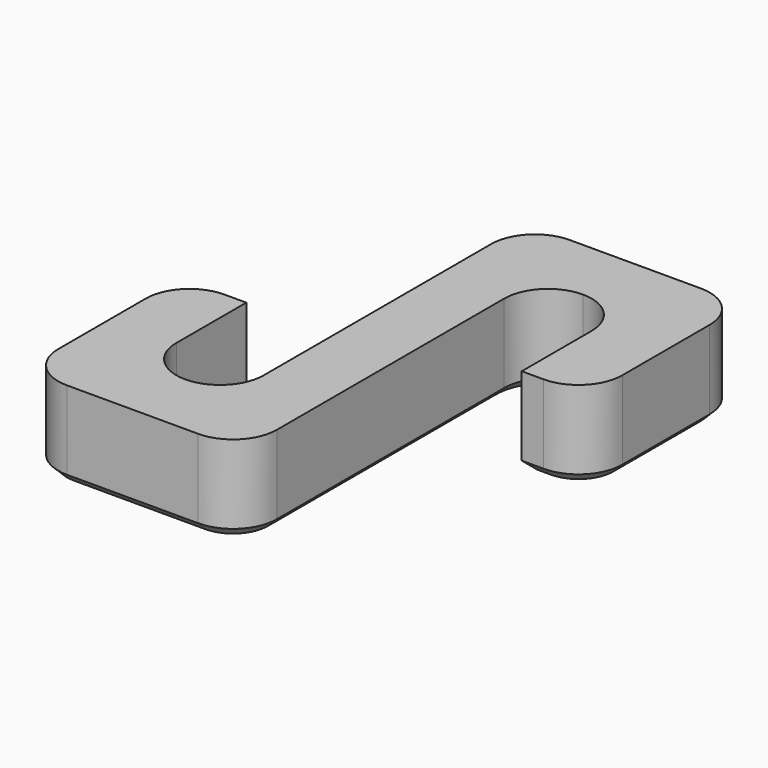
from build123d import *

# Parameters (mm, degrees)
F1_DEPTH = 2
F2_R     = 0.99999
F3_SIZE  = 0.2


# Not quite as in the source:
# - a fillet or chamfer is up to 0.001 mm smaller than in the source, because OpenCascade refuses the exact size


with BuildPart() as f1:
    # F0 (on Top) → F1 (new body)
    with BuildSketch(Plane.XY):
        Polygon((-0.75, 5), (-0.75, 0), (-0.75, -3.5), (-2.75, -3.5), (-2.75, -0.5), (-4.25, -0.5), (-4.25, -5), (0.75, -5), (0.75, 0), (0.75, 3.5), (2.75, 3.5), (2.75, 0.5), (4.25, 0.5), (4.25, 5), align=None)
    extrude(amount=F1_DEPTH)

    # F2 (radius 1 in the source; OpenCascade refuses exactly that, so slightly less here)
    f2_edges = [f1.edges().sort_by_distance(p)[0] for p in [
        (-0.75, 5, 1),
        (0.75, 3.5, 1),
        (2.75, 3.5, 1),
        (4.25, 5, 1),
        (4.25, 0.5, 1),
        (0.75, -5, 1),
        (-4.25, -5, 1),
        (-4.25, -0.5, 1),
        (-0.75, -3.5, 1),
        (-2.75, -3.5, 1),
    ]]
    fillet(f2_edges, radius=F2_R)

    # F3
    f3_edges = [f1.edges().sort_by_distance(p)[0] for p in [
        (-0.75, 0.75, 0),
        (-0.45711, 4.70711, 0),
        (-1.04289, -3.20711, 0),
        (1.75, 5, 0),
        (-1.75, -3.5, 0),
        (3.95711, 4.70711, 0),
        (-2.45711, -3.20711, 0),
        (4.25, 2.75, 0),
        (-2.75, -1.500005, 0),
        (3.95711, 0.79289, 0),
        (-3.000005, -0.5, 0),
        (3.000005, 0.5, 0),
        (-3.95711, -0.79289, 0),
        (2.75, 1.500005, 0),
        (-4.25, -2.75, 0),
        (2.45711, 3.20711, 0),
        (-3.95711, -4.70711, 0),
        (1.75, 3.5, 0),
        (-1.75, -5, 0),
        (1.04289, 3.20711, 0),
        (0.45711, -4.70711, 0),
        (0.75, -0.75, 0),
    ]]
    chamfer(f3_edges, length=F3_SIZE)


solid = f1.part
